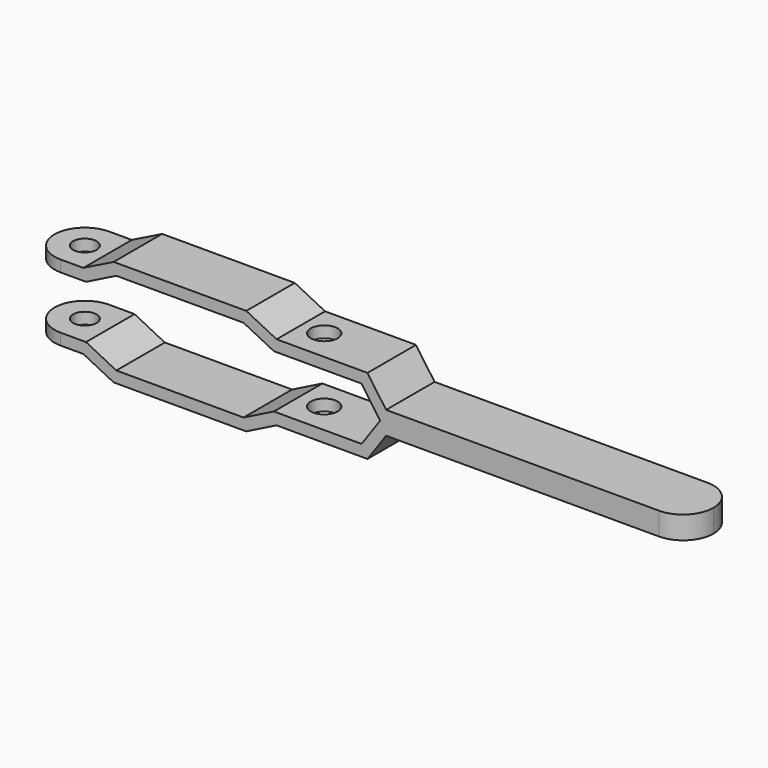
from build123d import *

# Parameters (mm, degrees)
F1_DEPTH    = 16
F2_T        = 3
F2_T3_DEPTH = 22
F3_R        = 7.99999
F4_R        = 3.1035458613
F4_R_2      = 3.5498541614
F5_DEPTH    = 20


# Not quite as in the source:
# - a fillet or chamfer is up to 0.001 mm smaller than in the source, because OpenCascade refuses the exact size
# - a shell that OpenCascade refuses in one call is made with other operations: the cavity is built on its own and cut out


with BuildPart() as f1:
    # F0 (on Front) → F1 (new body)
    with BuildSketch(Plane.XZ):
        Polygon((-64.2090581298, 10), (-64.2090581298, 0), (31.7909418702, 0), (29.6909418702, 3), (24.7909418702, 10), (0.7909418702, 10), (-7.2090581298, 14), (-42.2090581298, 14), (-50.2090581298, 10), align=None)
        Polygon((31.7909418702, 0), (-64.2090581298, 0), (-64.2090581298, -10), (-50.2090581298, -10), (-42.2090581298, -14), (-7.2090581298, -14), (0.7909418702, -10), (24.7909418702, -10), (29.6909418702, -3), align=None)
        Polygon((29.6909418702, 3), (31.7909418702, 0), (29.6909418702, -3), (109.6909418702, -3), (109.6909418702, 3), align=None)
    extrude(amount=F1_DEPTH)

    # F2: shell of thickness 3, made by hand


with BuildPart() as f2_core1:
    # F2_t2: copy of F1
    add(f1.part)

    # the walls: a layer under each face that stays
    f2_faces = [f2_core1.faces().sort_by_distance(p)[0] for p in [
        (-24.7090581298, -8, 14),
        (-46.2090581298, -8, 12),
        (-57.2090581298, -8, 10),
        (-57.2090581298, -8, -10),
        (-46.2090581298, -8, -12),
        (-24.7090581298, -8, -14),
        (-3.2090581298, -8, -12),
        (12.7909418702, -8, -10),
        (27.2409418702, -8, -6.5),
        (69.6909418702, -8, -3),
        (109.6909418702, -8, 0),
        (69.6909418702, -8, 3),
        (27.2409418702, -8, 6.5),
        (12.7909418702, -8, 10),
        (-3.2090581298, -8, 12),
    ]]
    thicken(f2_faces, amount=-F2_T, mode=Mode.SUBTRACT)

    # F2_s4 → F2_t3 (cut)
    with BuildSketch(Plane.XZ.offset(-3)):
        Polygon((-50.2224745377, 10.0568328157), (-48.8674173433, 7.316718427), (-49.5008541973, 7), (-50.2090581298, 7), align=None)
        Polygon((-50.2224745377, -10.0568328157), (-50.2090581298, -7), (-49.5008541973, -7), (-48.8674173433, -7.316718427), align=None)
        Polygon((0.8043582781, -10.0568328157), (-0.5506989163, -7.316718427), (0.0827379377, -7), (0.7909418702, -7), align=None)
        Polygon((29.7155188278, -3.0472038703), (27.2332461087, -1.2796129669), (28.1289751855, 0), (29.6909418702, 0), align=None)
        Polygon((29.7155188278, 3.0472038703), (29.6909418702, 0), (28.1289751855, 0), (27.2332461087, 1.2796129669), align=None)
        Polygon((0.8043582781, 10.0568328157), (0.7909418702, 7), (0.0827379377, 7), (-0.5506989163, 7.316718427), align=None)
    extrude(amount=F2_T3_DEPTH, mode=Mode.SUBTRACT)


with BuildPart() as f1_1:
    add(f1.part)

    # what is left inside the walls is the cavity
    f2_cavity = [f2_core1.part.solids().sort_by_distance(p)[0] for p in [
        (-18.040041, -15.97, -3.666667),
    ]]
    add(f2_cavity, mode=Mode.SUBTRACT)

    # F3 (radius 8 in the source; OpenCascade refuses exactly that, so slightly less here)
    f3_edges = [f1_1.edges().sort_by_distance(p)[0] for p in [
        (-64.209058, -16, -8.5),
        (-64.209058, -16, 8.5),
        (-64.209058, 0, -8.5),
        (-64.209058, 0, 8.5),
        (109.690942, -16, 0),
        (109.690942, 0, 0),
    ]]
    fillet(f3_edges, radius=F3_R)

    # F4 (on face) → F5 (cut)
    with BuildSketch(Plane.XY.offset(10)):
        with Locations((-56.2090581298, -8)):
            Circle(F4_R)
        with Locations((6.7909418702, -7.7808454374)):
            Circle(F4_R_2)
    extrude(amount=-F5_DEPTH, mode=Mode.SUBTRACT)


solid = f1_1.part
